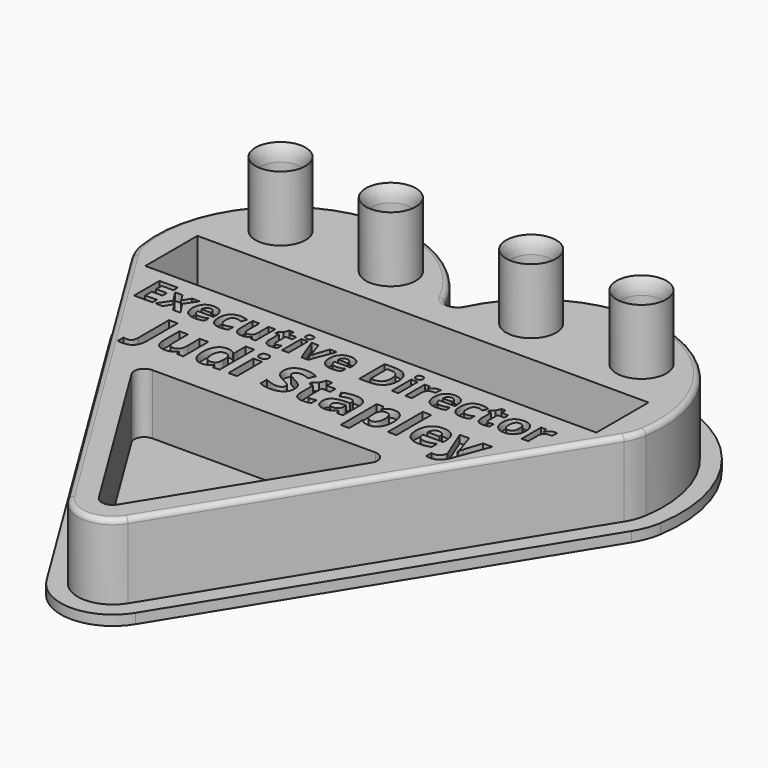
from build123d import *

# Parameters (mm, degrees)
F1_DEPTH       = 15
F2_W           = 90
F2_H           = 13
F2_R           = 5
F3_DEPTH       = 12
F5_DEPTH       = 2
F6_R           = 5
F6_R_2         = 4
F7_DEPTH       = 25
F8_TEXT_SIZE   = 8.8829504027
F8_TEXT_SIZE_2 = 11.4201949318
F9_DEPTH       = 1.5
F10_R          = 1


# Not quite as in the source:
# - a fillet or chamfer that OpenCascade refuses, or shapes differently, is made with other operations: its cross-section is extruded or revolved along the edge and cut away or added
# - Text() gives the source's letters only with a copy of the font that has no kerning and outlines rounded to 1/6400 em; it was checked with that copy


with BuildPart() as f1:
    # F0 (on Top) → F1 (new body)
    with BuildSketch(Plane.XY):
        with BuildLine():
            ThreePointArc((-5.95618879, -71.3351756816), (0, -74.6577016711), (5.95618879, -71.3351756816))
            Line((5.95618879, -71.3351756816), (49.0848252654, -1.4822547977))
            ThreePointArc((49.0848252654, -1.4822547977), (49.9475095022, 0.2820801212), (50.4487244655, 2.1809970121))
            ThreePointArc((50.4487244655, 2.1809970121), (32.7486654237, 30.8647670325), (1.800066042, 17.5143007867))
            ThreePointArc((1.800066042, 17.5143007867), (0, 16.3859442026), (-1.800066042, 17.5143007867))
            ThreePointArc((-1.800066042, 17.5143007867), (-32.7486654237, 30.8647670325), (-50.4487244655, 2.1809970121))
            ThreePointArc((-50.4487244655, 2.1809970121), (-49.9475095022, 0.2820801212), (-49.0848252654, -1.4822547977))
            Line((-49.0848252654, -1.4822547977), (-5.95618879, -71.3351756816))
        make_face()
    extrude(amount=F1_DEPTH)

    # F2 (on face) → F3 (cut)
    with BuildSketch(Plane.XY.offset(15)):
        with Locations((-0.0512755345, 3.2490186568)):
            Rectangle(F2_W, F2_H)
        with Locations((-36, 19.1686091315)):
            Circle(F2_R)
        with Locations((-14, 19.1686091315)):
            Circle(F2_R)
        with Locations((14, 19.1686091315)):
            Circle(F2_R)
        with Locations((36, 19.1686091315)):
            Circle(F2_R)
        with BuildLine():
            ThreePointArc((-1.8719450382, -68.813479211), (0, -69.8577016592), (1.8719450382, -68.813479211))
            Line((1.8719450382, -68.813479211), (23.9552123995, -33.0465073353))
            ThreePointArc((23.9552123995, -33.0465073353), (24.0000714552, -31.0214837198), (22.2534441738, -29.9958004752))
            Line((22.2534441738, -29.9958004752), (-22.2534441738, -29.9958004752))
            ThreePointArc((-22.2534441738, -29.9958004752), (-24.0000714552, -31.0214837198), (-23.9552123995, -33.0465073353))
            Line((-23.9552123995, -33.0465073353), (-1.8719450382, -68.813479211))
        make_face()
    extrude(amount=-F3_DEPTH, mode=Mode.SUBTRACT)

    # F4 (on face) → F5 (join)
    with BuildSketch(Plane(origin=(0, 0, 0), x_dir=(1, 0, 0), z_dir=(0, 0, -1))):
        with BuildLine():
            Line((-8.8491942253, 73.1213770052), (-51.9778307007, 3.2684561212))
            ThreePointArc((-51.9778307007, 3.2684561212), (-53.1338275223, 0.9042474437), (-53.8054555409, -1.6403010677))
            ThreePointArc((-53.8054555409, -1.6403010677), (-35.0235705821, -33.6811648353), (0, -21.3229425821))
            ThreePointArc((0, -21.3229425821), (35.0235705821, -33.6811648353), (53.8054555409, -1.6403010677))
            ThreePointArc((53.8054555409, -1.6403010677), (53.1338275223, 0.9042474437), (51.9778307007, 3.2684561212))
            Line((51.9778307007, 3.2684561212), (8.8491942253, 73.1213770052))
            ThreePointArc((8.8491942253, 73.1213770052), (0, 78.0577010266), (-8.8491942253, 73.1213770052))
        make_face()
    extrude(amount=F5_DEPTH)

    # F6 (on face) → F7 (join)
    with BuildSketch(Plane.XY.offset(3)):
        with Locations((-14, 19.1686091315)):
            Circle(F6_R)
        with Locations((-14, 19.1686091315)):
            Circle(F6_R_2, mode=Mode.SUBTRACT)
        with Locations((14, 19.1686091315)):
            Circle(F6_R)
        with Locations((14, 19.1686091315)):
            Circle(F6_R_2, mode=Mode.SUBTRACT)
        with Locations((36, 19.1686091315)):
            Circle(F6_R)
        with Locations((36, 19.1686091315)):
            Circle(F6_R_2, mode=Mode.SUBTRACT)
        with Locations((-36, 19.1686091315)):
            Circle(F6_R)
        with Locations((-36, 19.1686091315)):
            Circle(F6_R_2, mode=Mode.SUBTRACT)
    extrude(amount=F7_DEPTH)

    # F8 (on face) → F9 (cut)
    with BuildSketch(Plane.XY.offset(15)):
        with Locations((-40.9787755345, -12.1467056332)):
            Text('Executive Director', F8_TEXT_SIZE, font='Open Sans', font_style=FontStyle.BOLD, text_align=(TextAlign.LEFT, TextAlign.BOTTOM))
        with Locations((-31.7787755345, -23.369245984)):
            Text('Judi Stapley', F8_TEXT_SIZE_2, font='Open Sans', font_style=FontStyle.BOLD, text_align=(TextAlign.LEFT, TextAlign.BOTTOM))
    extrude(amount=-F9_DEPTH, mode=Mode.SUBTRACT)

    # F10
    f10_edges = [f1.edges().sort_by_distance(p)[0] for p in [
        (32.748665, 30.864767, 15),
        (49.94751, 0.28208, 15),
        (27.520507, -36.408715, 15),
        (0, -74.657702, 15),
        (-27.520507, -36.408715, 15),
        (-32.748665, 30.864767, 15),
        (-49.94751, 0.28208, 15),
        (0, 16.385944, 15),
    ]]
    fillet(f10_edges, radius=F10_R)

    # F11: fillet of radius 5 on 4 edges, made by hand

    # F11_s1 → F11_t2 (revolve, cut)
    with BuildSketch(Plane.XZ.offset(-19.1686091315)):
        with BuildLine():
            ThreePointArc((-31, 28), (-31.7434164903, 26.5811388301), (-32, 25))
            Line((-32, 25), (-32, 28))
            Line((-32, 28), (-31, 28))
        make_face()
    revolve(axis=Axis((-36, 19.1686091315, 28), (0, 0, 1)), mode=Mode.SUBTRACT)

    # F11_s3 → F11_t4 (revolve, cut)
    with BuildSketch(Plane.XZ.offset(-19.1686091315)):
        with BuildLine():
            ThreePointArc((-9, 28), (-9.7434164903, 26.5811388301), (-10, 25))
            Line((-10, 25), (-10, 28))
            Line((-10, 28), (-9, 28))
        make_face()
    revolve(axis=Axis((-14, 19.1686091315, 28), (0, 0, 1)), mode=Mode.SUBTRACT)

    # F11_s5 → F11_t6 (revolve, cut)
    with BuildSketch(Plane.XZ.offset(-19.1686091315)):
        with BuildLine():
            ThreePointArc((19, 28), (18.2565835097, 26.5811388301), (18, 25))
            Line((18, 25), (18, 28))
            Line((18, 28), (19, 28))
        make_face()
    revolve(axis=Axis((14, 19.1686091315, 28), (0, 0, 1)), mode=Mode.SUBTRACT)

    # F11_s7 → F11_t8 (revolve, cut)
    with BuildSketch(Plane.XZ.offset(-19.1686091315)):
        with BuildLine():
            ThreePointArc((41, 28), (40.2565835097, 26.5811388301), (40, 25))
            Line((40, 25), (40, 28))
            Line((40, 28), (41, 28))
        make_face()
    revolve(axis=Axis((36, 19.1686091315, 28), (0, 0, 1)), mode=Mode.SUBTRACT)


solid = f1.part
